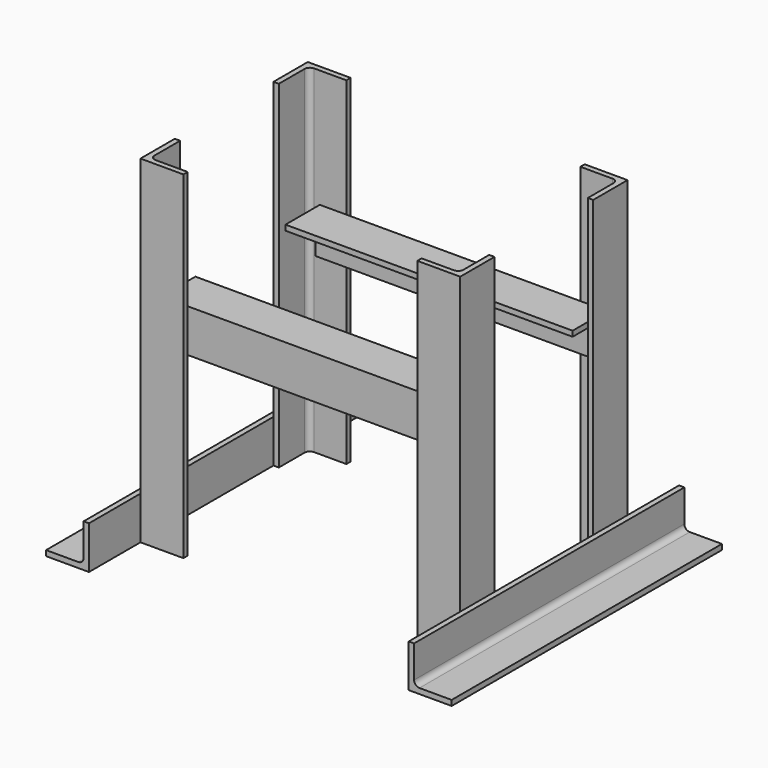
from build123d import *

# Parameters (mm, degrees)
F1_DEPTH = 200
F3_DEPTH = 400
F6_DEPTH = 170


# Not quite as in the source:
# - a pattern or mirror of a feature is missing from the dataset's text; its kind, count and spacing are read off the source's solid


with BuildPart() as f1:
    # F0 (on Front) → F1 (new body, symmetric)
    with BuildSketch(Plane.XZ):
        with BuildLine():
            Line((-240.1, 0), (-189.3, 0))
            Line((-189.3, 0), (-189.3, 50.8))
            Line((-189.3, 50.8), (-195.65, 50.8))
            Line((-195.65, 50.8), (-195.65, 12.7))
            ThreePointArc((-195.65, 12.7), (-197.5098719395, 8.2098719395), (-202, 6.35))
            Line((-202, 6.35), (-240.1, 6.35))
            Line((-240.1, 6.35), (-240.1, 0))
        make_face()
    extrude(amount=F1_DEPTH, both=True)

    # F2 (on Top) → F3 (join)
    with BuildSketch(Plane.XY):
        with BuildLine():
            Line((-138.5, 123.8), (-189.3, 123.8))
            Line((-189.3, 123.8), (-189.3, 73))
            Line((-189.3, 73), (-182.95, 73))
            Line((-182.95, 73), (-182.95, 111.1))
            ThreePointArc((-182.95, 111.1), (-181.0901280605, 115.5901280605), (-176.6, 117.45))
            Line((-176.6, 117.45), (-138.5, 117.45))
            Line((-138.5, 117.45), (-138.5, 123.8))
        make_face()
    f3 = extrude(amount=F3_DEPTH)

    # F3_copies: F3 across plane
    add(f3.mirror(Plane(origin=(0, 0, 0), x_dir=(0, 0, -1), z_dir=(0, -1, 0))))


with BuildPart() as f4_1:
    # F4: instance of F1
    add(f1.part.mirror(Plane.YZ))


with BuildPart() as f6:
    # F5 (on Right) → F6 (new body, symmetric)
    with BuildSketch(Plane.YZ):
        with BuildLine():
            Line((-66.65, 260), (-117.45, 260))
            Line((-117.45, 260), (-117.45, 209.2))
            Line((-117.45, 209.2), (-111.1, 209.2))
            Line((-111.1, 209.2), (-111.1, 247.3))
            ThreePointArc((-111.1, 247.3), (-109.2401280605, 251.7901280605), (-104.75, 253.65))
            Line((-104.75, 253.65), (-66.65, 253.65))
            Line((-66.65, 253.65), (-66.65, 260))
        make_face()
    extrude(amount=F6_DEPTH, both=True)


with BuildPart() as f7_1:
    # F7: instance of F6
    add(f6.part.mirror(Plane.XZ))


solid = Compound([f1.part, f4_1.part, f6.part, f7_1.part])
